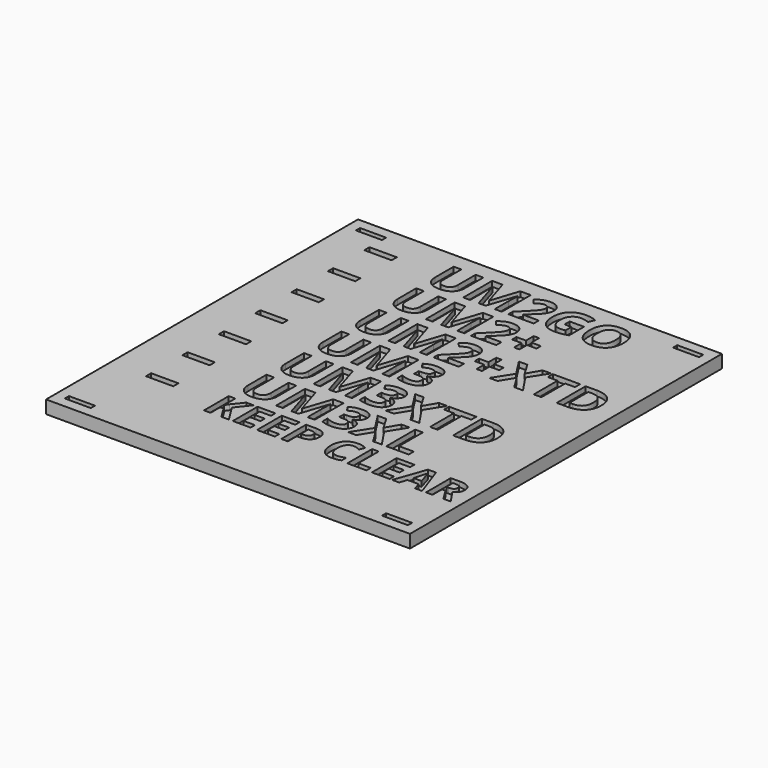
from build123d import *

# Parameters (mm, degrees)
F0_W           = 140
F0_H           = 150
F1_DEPTH       = 5
F2_TEXT_SIZE   = 19.4444444444
F2_TEXT_SIZE_2 = 16.6666666667
F3_DEPTH       = 2
F4_W           = 10.5
F4_H           = 2.5
F4_W_2         = 10
F4_H_2         = 2
F5_DEPTH       = 25


# Not quite as in the source:
# - Text() gives the source's letters only with a copy of the font that has no kerning and outlines rounded to 1/6400 em; it was checked with that copy


with BuildPart() as f1:
    # F0 (on Top) → F1 (new body)
    with BuildSketch(Plane.XY):
        with Locations((19.2060028017, -10.4792832956)):
            Rectangle(F0_W, F0_H)
    extrude(amount=F1_DEPTH)

    # F2 (on face) → F3 (cut)
    with BuildSketch(Plane.XY.offset(5)):
        with Locations((-10.7939971983, 44.5921175071)):
            Text('UM2GO', F2_TEXT_SIZE, font='Open Sans', font_style=FontStyle.BOLD, text_align=(TextAlign.LEFT, TextAlign.BOTTOM))
        with Locations((-10.7939971983, 26.5921175071)):
            Text('UM2+', F2_TEXT_SIZE, font='Open Sans', font_style=FontStyle.BOLD, text_align=(TextAlign.LEFT, TextAlign.BOTTOM))
        with Locations((-10.7939971983, 8.5921175071)):
            Text('UM2+XTD', F2_TEXT_SIZE, font='Open Sans', font_style=FontStyle.BOLD, text_align=(TextAlign.LEFT, TextAlign.BOTTOM))
        with Locations((-10.7939971983, -9.4078824929)):
            Text('UM3', F2_TEXT_SIZE, font='Open Sans', font_style=FontStyle.BOLD, text_align=(TextAlign.LEFT, TextAlign.BOTTOM))
        with Locations((-10.7939971983, -27.4078824929)):
            Text('UM3XTD', F2_TEXT_SIZE, font='Open Sans', font_style=FontStyle.BOLD, text_align=(TextAlign.LEFT, TextAlign.BOTTOM))
        with Locations((-10.7939971983, -45.4078824929)):
            Text('UM3XL', F2_TEXT_SIZE, font='Open Sans', font_style=FontStyle.BOLD, text_align=(TextAlign.LEFT, TextAlign.BOTTOM))
        with Locations((-10.7939971983, -61.4078824929)):
            Text('KEEP CLEAR', F2_TEXT_SIZE_2, font='Open Sans', font_style=FontStyle.BOLD, text_align=(TextAlign.LEFT, TextAlign.BOTTOM))
    extrude(amount=-F3_DEPTH, mode=Mode.SUBTRACT)

    # F4 (on face) → F5 (cut)
    with BuildSketch(Plane.XY.offset(5)):
        with Locations((-31.5439971983, 51.3051763475)):
            Rectangle(F4_W, F4_H)
        with Locations((-31.5439971983, 33.8051763475)):
            Rectangle(F4_W, F4_H)
        with Locations((-31.5439971983, 16.3051763475)):
            Rectangle(F4_W, F4_H)
        with Locations((-31.5439971983, -1.1948236525)):
            Rectangle(F4_W, F4_H)
        with Locations((-31.5439971983, -18.6948236525)):
            Rectangle(F4_W, F4_H)
        with Locations((-31.5439971983, -36.1948236525)):
            Rectangle(F4_W, F4_H)
        with Locations((-31.5439971983, -53.6948236525)):
            Rectangle(F4_W, F4_H)
        with Locations((80.2060028017, -80.4792832956)):
            Rectangle(F4_W_2, F4_H_2)
        with Locations((-41.7939971983, 59.5207167044)):
            Rectangle(F4_W_2, F4_H_2)
        with Locations((-41.7939971983, -80.4792832956)):
            Rectangle(F4_W_2, F4_H_2)
        with Locations((-61.5124900618, -96.4436668555)):
            Rectangle(F4_W_2, F4_H_2)
        with Locations((-32.1325899826, -118.0590648154)):
            Rectangle(F4_W_2, F4_H_2)
        with Locations((16.2765893361, -117.943051825)):
            Rectangle(F4_W_2, F4_H_2)
        with Locations((80.2060028017, 59.5207167044)):
            Rectangle(F4_W_2, F4_H_2)
        with Locations((-41.7294901609, 200.6763165593)):
            Rectangle(F4_W_2, F4_H_2)
    extrude(amount=-F5_DEPTH, mode=Mode.SUBTRACT)


solid = f1.part
